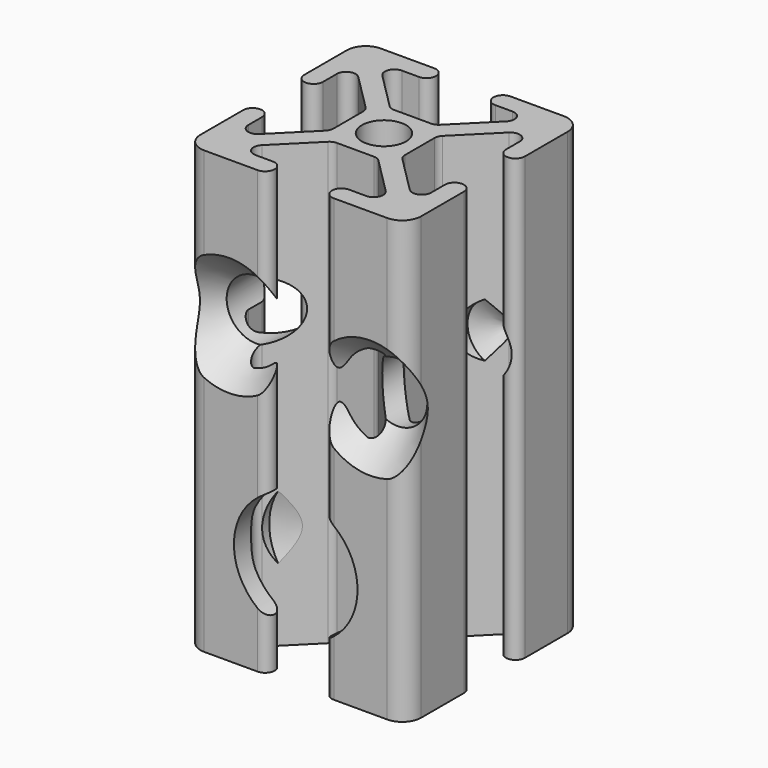
from build123d import *

# Parameters (mm, degrees)
F0_R           = 2.5
F1_DEPTH       = 50
F3_D           = 6.7564
F3_DEPTH       = 18
F3_CSINK_D     = 13.4874
F3_CSINK_ANGLE = 82
F3_TIP         = 2.0298273432
F5_D           = 14
F5_DEPTH       = 5
F5_TIP         = 4.2060243332


with BuildPart() as f1:
    # F0 (on Top) → F1 (new body)
    with BuildSketch(Plane.XY):
        with BuildLine():
            ThreePointArc((-10.36, 12.5), (-11.8732085117, 11.8732085117), (-12.5, 10.36))
            Line((-12.5, 10.36), (-12.5, 4.32))
            ThreePointArc((-12.5, 4.32), (-11.43, 3.25), (-10.36, 4.32))
            Line((-10.36, 4.32), (-10.36, 6.2635829765))
            ThreePointArc((-10.36, 6.2635829765), (-9.6994712726, 7.2521340763), (-8.5333957441, 7.0201872324))
            Line((-8.5333957441, 7.0201872324), (-4.3633957441, 2.8501872324))
            ThreePointArc((-4.3633957441, 2.8501872324), (-4.1314489002, 2.5030542492), (-4.05, 2.0935829765))
            Line((-4.05, 2.0935829765), (-4.05, 0))
            Line((-4.05, 0), (-4.05, -2.0935829765))
            ThreePointArc((-4.05, -2.0935829765), (-4.1314489002, -2.5030542492), (-4.3633957441, -2.8501872324))
            Line((-4.3633957441, -2.8501872324), (-8.5333957441, -7.0201872324))
            ThreePointArc((-8.5333957441, -7.0201872324), (-9.6994712726, -7.2521340763), (-10.36, -6.2635829765))
            Line((-10.36, -6.2635829765), (-10.36, -4.32))
            ThreePointArc((-10.36, -4.32), (-11.43, -3.25), (-12.5, -4.32))
            Line((-12.5, -4.32), (-12.5, -10.36))
            ThreePointArc((-12.5, -10.36), (-11.8732085117, -11.8732085117), (-10.36, -12.5))
            Line((-10.36, -12.5), (-4.32, -12.5))
            ThreePointArc((-4.32, -12.5), (-3.25, -11.43), (-4.32, -10.36))
            Line((-4.32, -10.36), (-6.2635829765, -10.36))
            ThreePointArc((-6.2635829765, -10.36), (-7.2521340763, -9.6994712726), (-7.0201872324, -8.5333957441))
            Line((-7.0201872324, -8.5333957441), (-2.8501872324, -4.3633957441))
            ThreePointArc((-2.8501872324, -4.3633957441), (-2.5030542492, -4.1314489002), (-2.0935829765, -4.05))
            Line((-2.0935829765, -4.05), (0, -4.05))
            Line((0, -4.05), (2.0935829765, -4.05))
            ThreePointArc((2.0935829765, -4.05), (2.5030542492, -4.1314489002), (2.8501872324, -4.3633957441))
            Line((2.8501872324, -4.3633957441), (7.0201872324, -8.5333957441))
            ThreePointArc((7.0201872324, -8.5333957441), (7.2521340763, -9.6994712726), (6.2635829765, -10.36))
            Line((6.2635829765, -10.36), (4.32, -10.36))
            ThreePointArc((4.32, -10.36), (3.25, -11.43), (4.32, -12.5))
            Line((4.32, -12.5), (10.36, -12.5))
            ThreePointArc((10.36, -12.5), (11.8732085117, -11.8732085117), (12.5, -10.36))
            Line((12.5, -10.36), (12.5, -4.32))
            ThreePointArc((12.5, -4.32), (11.43, -3.25), (10.36, -4.32))
            Line((10.36, -4.32), (10.36, -6.2635829765))
            ThreePointArc((10.36, -6.2635829765), (9.6994712726, -7.2521340763), (8.5333957441, -7.0201872324))
            Line((8.5333957441, -7.0201872324), (4.3633957441, -2.8501872324))
            ThreePointArc((4.3633957441, -2.8501872324), (4.1314489002, -2.5030542492), (4.05, -2.0935829765))
            Line((4.05, -2.0935829765), (4.05, 0))
            Line((4.05, 0), (4.05, 2.0935829765))
            ThreePointArc((4.05, 2.0935829765), (4.1314489002, 2.5030542492), (4.3633957441, 2.8501872324))
            Line((4.3633957441, 2.8501872324), (8.5333957441, 7.0201872324))
            ThreePointArc((8.5333957441, 7.0201872324), (9.6994712726, 7.2521340763), (10.36, 6.2635829765))
            Line((10.36, 6.2635829765), (10.36, 4.32))
            ThreePointArc((10.36, 4.32), (11.43, 3.25), (12.5, 4.32))
            Line((12.5, 4.32), (12.5, 10.36))
            ThreePointArc((12.5, 10.36), (11.8732085117, 11.8732085117), (10.36, 12.5))
            Line((10.36, 12.5), (4.32, 12.5))
            ThreePointArc((4.32, 12.5), (3.25, 11.43), (4.32, 10.36))
            Line((4.32, 10.36), (6.2635829765, 10.36))
            ThreePointArc((6.2635829765, 10.36), (7.2521340763, 9.6994712726), (7.0201872324, 8.5333957441))
            Line((7.0201872324, 8.5333957441), (2.8501872324, 4.3633957441))
            ThreePointArc((2.8501872324, 4.3633957441), (2.5030542492, 4.1314489002), (2.0935829765, 4.05))
            Line((2.0935829765, 4.05), (0, 4.05))
            Line((0, 4.05), (-2.0935829765, 4.05))
            ThreePointArc((-2.0935829765, 4.05), (-2.5030542492, 4.1314489002), (-2.8501872324, 4.3633957441))
            Line((-2.8501872324, 4.3633957441), (-7.0201872324, 8.5333957441))
            ThreePointArc((-7.0201872324, 8.5333957441), (-7.2521340763, 9.6994712726), (-6.2635829765, 10.36))
            Line((-6.2635829765, 10.36), (-4.32, 10.36))
            ThreePointArc((-4.32, 10.36), (-3.25, 11.43), (-4.32, 12.5))
            Line((-4.32, 12.5), (-10.36, 12.5))
        make_face()
        Circle(F0_R, mode=Mode.SUBTRACT)
    extrude(amount=F1_DEPTH)

    # F3
    with Locations(Plane.XZ.offset(12.5)):
        with Locations((-7.5452360325, 33.4570966661), (8.4325838834, 30.4279308766)):
            CounterSinkHole(F3_D / 2, F3_CSINK_D / 2, depth=F3_DEPTH, counter_sink_angle=F3_CSINK_ANGLE)
            with Locations((0, 0, -(F3_DEPTH + F3_TIP / 2))):  # 118° drill point
                Cone(0, F3_D / 2, F3_TIP, mode=Mode.SUBTRACT)

    # F5 (one way)
    with BuildSketch(Plane.XZ.offset(12.5)):
        with Locations((0, 11.8282912299)):
            Circle(F5_D / 2)
    extrude(amount=-F5_DEPTH, mode=Mode.SUBTRACT)
    with Locations(Plane.XZ.offset(12.5)):
        with Locations((0, 11.8282912299)):
            with Locations((0, 0, -(F5_DEPTH + F5_TIP / 2))):  # 118° drill point
                Cone(0, F5_D / 2, F5_TIP, mode=Mode.SUBTRACT)


solid = f1.part
